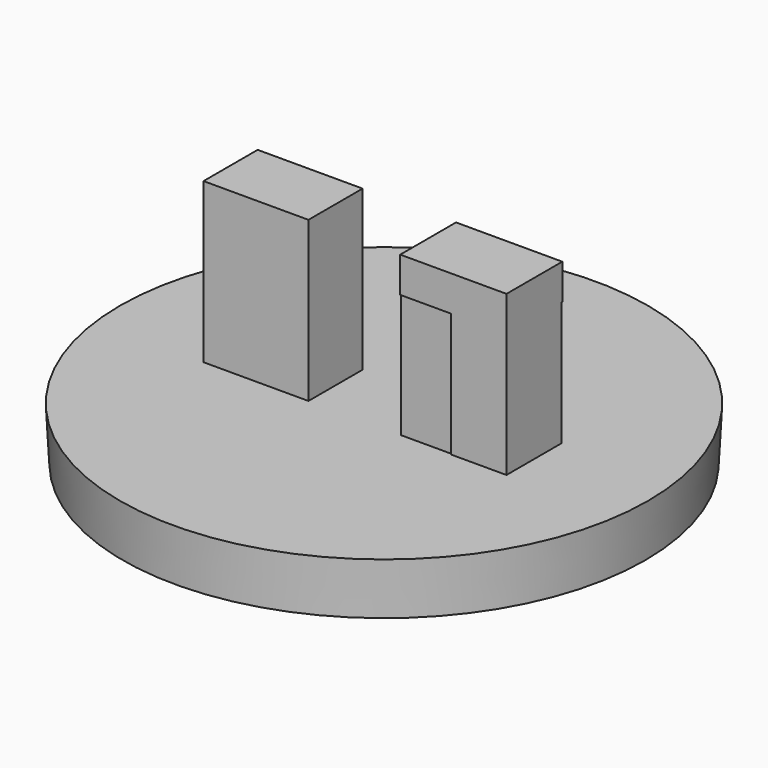
from build123d import *

# Parameters (mm, degrees)
F0_R     = 14.7481793899
F1_DEPTH = 3
F1_TAPER = -3
F2_W     = 2.8173960745
F2_H     = 3.8187131286
F2_W_2   = 2.8887987137
F3_DEPTH = 7
F4_W     = 5.9206429869
F4_H     = 3.8187131286
F4_W_2   = 5.9958791826
F4_H_2   = 3.9352546446
F5_DEPTH = 2
F6_W     = 3.1207427382
F6_H     = 3.8840055931
F7_DEPTH = 7
F8_W     = 3.1032469124
F8_H     = 3.8187131286
F9_DEPTH = 7


with BuildPart() as f1:
    # F0 (on Top) → F1 (new body)
    with BuildSketch(Plane.XY):
        Circle(F0_R)
    extrude(amount=F1_DEPTH, taper=F1_TAPER)

    # F2 (on face) → F3 (join)
    with BuildSketch(Plane.XY.offset(3)):
        with Locations((-4.1453484446, 0)):
            Rectangle(F2_W, F2_H)
        with Locations((3.9267931134, 0)):
            Rectangle(F2_W_2, F2_H)
    extrude(amount=F3_DEPTH)

    # F4 (on face) → F5 (join)
    with BuildSketch(Plane.XY.offset(10)):
        with Locations((-5.6969719008, 0)):
            Rectangle(F4_W, F4_H)
        with Locations((5.4939956171, -0.0070217066)):
            Rectangle(F4_W_2, F4_H_2)
    extrude(amount=F5_DEPTH)

    # F6 (on face) → F7 (join)
    with BuildSketch(Plane(origin=(0, 0, 10), x_dir=(1, 0, 0), z_dir=(0, 0, -1))):
        with Locations((6.9315638393, 0.0326462323)):
            Rectangle(F6_W, F6_H)
    extrude(amount=F7_DEPTH)

    # F8 (on face) → F9 (join)
    with BuildSketch(Plane(origin=(0, 0, 10), x_dir=(1, 0, 0), z_dir=(0, 0, -1))):
        with Locations((-7.105669938, 0)):
            Rectangle(F8_W, F8_H)
    extrude(amount=F9_DEPTH)


solid = f1.part
